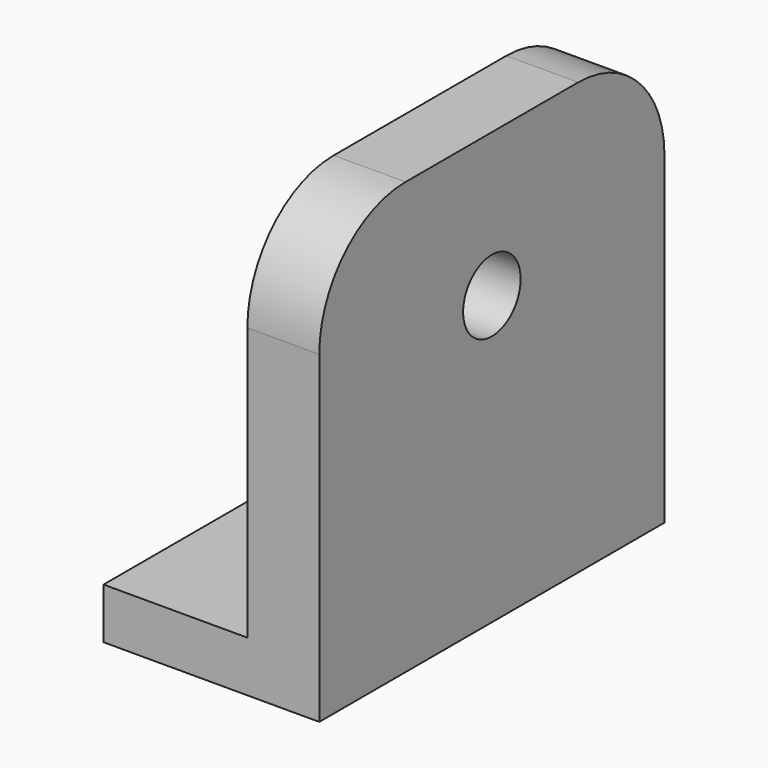
from build123d import *

# Parameters (mm, degrees)
F1_DEPTH = 76.2
F2_R     = 12.7
F3_DEPTH = 76.201
F5_DEPTH = 17.9342755506
F7_DEPTH = 25.401


# Not quite as in the source:
# - a pattern or mirror of a feature is missing from the dataset's text; its kind, count and spacing are read off the source's solid


with BuildPart() as f1:
    # F0 (on Front) → F1 (new body, symmetric)
    with BuildSketch(Plane.XZ):
        Polygon((0, 0), (0, 152.4), (-25.4, 152.4), (-25.4, 17.9332755506), (-76.2, 17.9332755506), (-76.2, 0), align=None)
    extrude(amount=F1_DEPTH, both=True)

    # F2 (on face) → F3 (cut, through all)
    with BuildSketch(Plane.YZ):
        with Locations((0, 101.6)):
            Circle(F2_R)
    extrude(amount=-F3_DEPTH, mode=Mode.SUBTRACT)

    # F4 (on face) → F5 (cut, through all)
    with BuildSketch(Plane.XY.offset(17.9332755506)):
        with BuildLine():
            Line((-63.5, 12.7), (-76.2, 12.7))
            Line((-76.2, 12.7), (-76.2, -12.7))
            Line((-76.2, -12.7), (-63.5, -12.7))
            ThreePointArc((-63.5, -12.7), (-50.8, 0), (-63.5, 12.7))
        make_face()
    extrude(amount=-F5_DEPTH, mode=Mode.SUBTRACT)

    # F6 (on face) → F7 (cut, through all)
    with BuildSketch(Plane(origin=(-25.4, 0, 0), x_dir=(0, -1, 0), z_dir=(-1, 0, 0))):
        with BuildLine():
            ThreePointArc((-76.2, 114.3), (-65.0407683632, 141.2407683632), (-38.1, 152.4))
            Line((-38.1, 152.4), (-76.2, 152.4))
            Line((-76.2, 152.4), (-76.2, 114.3))
        make_face()
    f7 = extrude(amount=-F7_DEPTH, mode=Mode.SUBTRACT)

    # F7_copies: F7 across plane
    add(f7.mirror(Plane(origin=(0, 0, 0), x_dir=(0, 0, -1), z_dir=(0, -1, 0))), mode=Mode.SUBTRACT)


solid = f1.part
